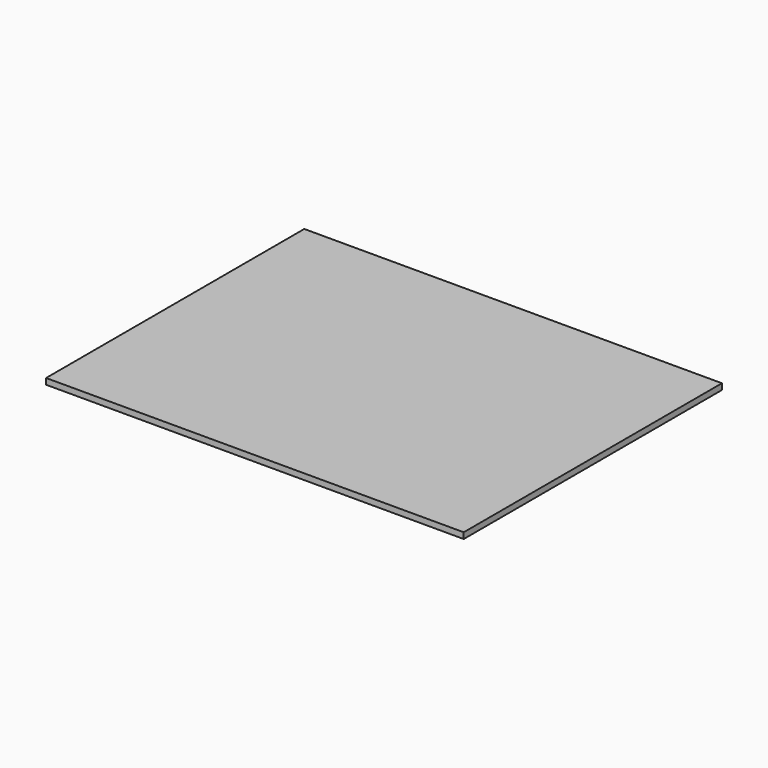
from build123d import *

# Parameters (mm, degrees)
F0_W     = 279.4
F0_H     = 215.9
F1_DEPTH = 4


# Not quite as in the source:
# - a feature names something its author has since deleted; it is built from what else it names


with BuildPart() as f1:
    # F0 (on Top) → F1 (new body)
    with BuildSketch(Plane.XY):
        Rectangle(F0_W, F0_H)
    extrude(amount=F1_DEPTH)


solid = f1.part
